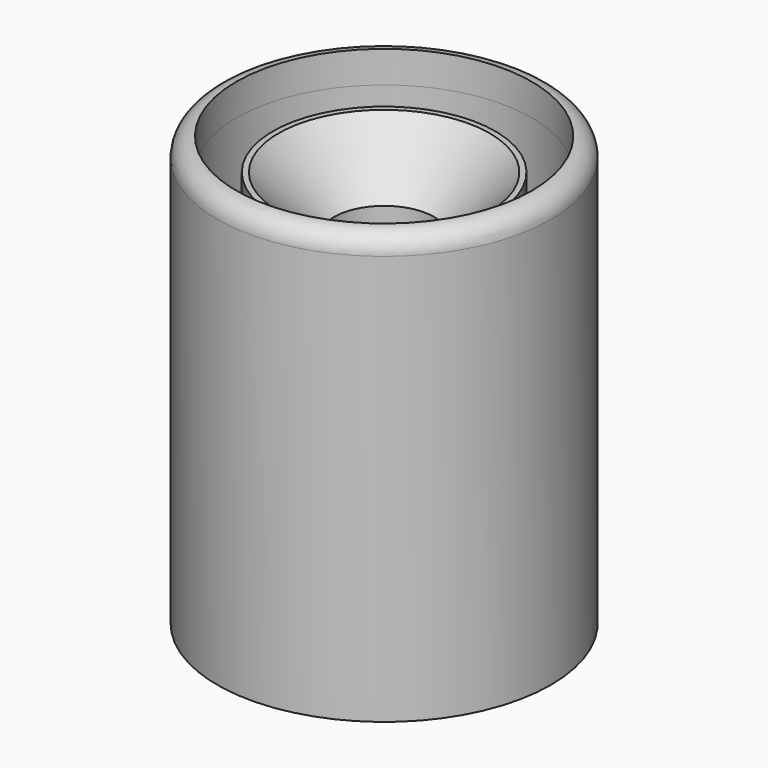
from build123d import *
from build123d import SkipClean  # not in build123d's __all__

# Parameters (mm, degrees)
F0_R     = 10.5
F0_R_2   = 3.15
F1_DEPTH = 25
F2_SIZE  = 3.5
F3_R     = 10.5
F3_R_2   = 9.3
F4_DEPTH = 2
F5_R     = 1.19999


# Not quite as in the source:
# - a fillet or chamfer is up to 0.001 mm smaller than in the source, because OpenCascade refuses the exact size


with BuildPart() as f1:
    # F0 (on Top) → F1 (new body)
    with BuildSketch(Plane.XY):
        Circle(F0_R)
        with BuildLine():
            ThreePointArc((2.678784, -6.467157), (0, 7), (-2.678784, -6.467157))
            Line((-2.678784, -6.467157), (-3.558956, -8.59208))
            ThreePointArc((-3.558956, -8.59208), (0, 9.3), (3.558956, -8.59208))
            Line((3.558956, -8.59208), (2.678784, -6.467157))
        make_face(mode=Mode.SUBTRACT)
        Circle(F0_R_2, mode=Mode.SUBTRACT)
    extrude(amount=F1_DEPTH)

    # F2
    f2_edges = [f1.edges().sort_by_distance(p)[0] for p in [
        (-3.15, 0, 25),
    ]]
    chamfer(f2_edges, length=F2_SIZE)

    # F3 (on face) → F4 (join)
    with BuildSketch(Plane.XY.offset(25)):
        Circle(F3_R)
        Circle(F3_R_2, mode=Mode.SUBTRACT)
    with SkipClean():  # cleaning this boolean's faces spoils the solid; the shape is the same uncleaned
        extrude(amount=F4_DEPTH)

    # F5 (radius 1.2 in the source; OpenCascade refuses exactly that, so slightly less here)
    f5_edges = [f1.edges().sort_by_distance(p)[0] for p in [
        (-10.5, 0, 27),
    ]]
    fillet(f5_edges, radius=F5_R)


solid = f1.part
